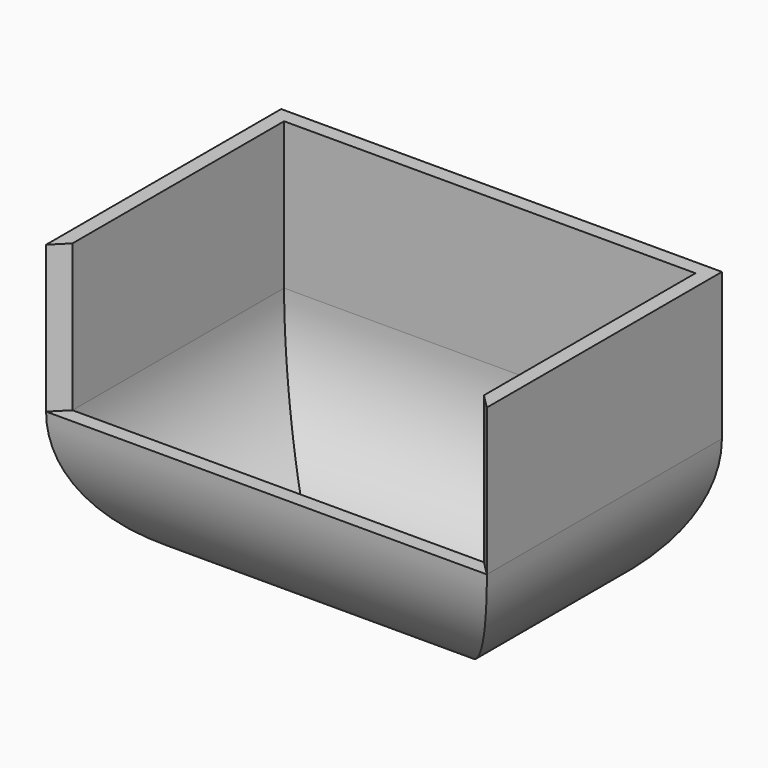
from build123d import *

# Parameters (mm, degrees)
F0_W     = 76.2
F0_H     = 50.8
F1_DEPTH = 25.4
F2_DEPTH = 25.4
F3_R     = 25.39999
F4_T     = -2.54
F6_D     = 3.81
F8_DEPTH = 25.4


# Not quite as in the source:
# - a fillet or chamfer is up to 0.001 mm smaller than in the source, because OpenCascade refuses the exact size


with BuildPart() as f1:
    # F0 (on Top) → F1 (new body)
    with BuildSketch(Plane.XY):
        Rectangle(F0_W, F0_H)
    extrude(amount=F1_DEPTH)

    # F2 (add): a face of the model
    f2_faces = [f1.faces().sort_by_distance(p)[0] for p in [
        (0, 0, 0),
    ]]
    extrude(f2_faces, amount=F2_DEPTH)

    # F3 (radius 25.4 in the source; OpenCascade refuses exactly that, so slightly less here)
    f3_edges = [f1.edges().sort_by_distance(p)[0] for p in [
        (0, -25.4, -25.4),
        (38.1, 0, -25.4),
        (0, 25.4, -25.4),
        (-38.1, 0, -25.4),
    ]]
    fillet(f3_edges, radius=F3_R)

    # F4
    f4_openings = [f1.faces().sort_by_distance(p)[0] for p in [
        (0, 0, 25.4),
    ]]
    offset(amount=F4_T, openings=f4_openings)

    # F6 (through all)
    with Locations(Plane.XY):
        with Locations((0, 0)):
            Hole(F6_D / 2)

    # F7 (on face) → F8 (cut)
    with BuildSketch(Plane.XY.offset(25.4)):
        Polygon((-35.56, -22.86), (-38.1, -25.4), (38.1, -25.4), (35.56, -22.86), align=None)
    extrude(amount=-F8_DEPTH, mode=Mode.SUBTRACT)


solid = f1.part
